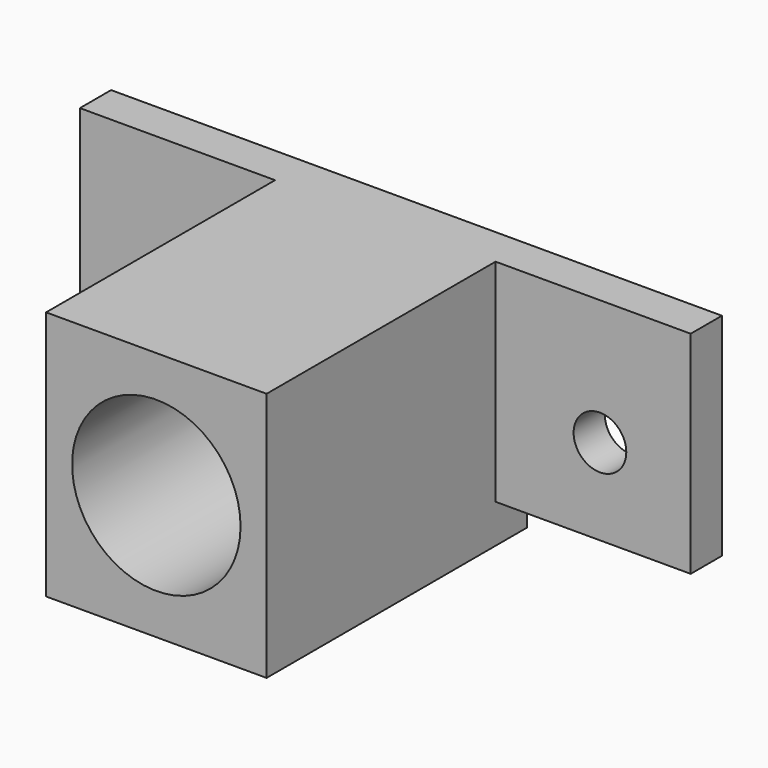
from build123d import *

# Parameters (mm, degrees)
F0_W         = 17.2212
F0_H         = 19.5351538889
F0_R         = 6.5786
F1_DEPTH     = 25.4
F2_W         = 15.24
F2_H         = 16.51
F2_R         = 2.0574
F3_DEPTH     = 3.048
F4_TEXT_SIZE = 2.3282805665
F5_DEPTH     = 22.86
F6_W         = 13.208
F6_H         = 11.43
F7_DEPTH     = 10.16


# Not quite as in the source:
# - a feature names something its author has since deleted; it is built from what else it names
# - Text() gives the source's letters only with a copy of the font that has no kerning and outlines rounded to 1/6400 em; it was checked with that copy


with BuildPart() as f1:
    # F0 (on Front) → F1 (new body)
    with BuildSketch(Plane.XZ):
        with Locations((-32.2175832933, 21.9545621703)):
            Rectangle(F0_W, F0_H)
        with Locations((-32.2175832933, 21.9405852258)):
            Circle(F0_R, mode=Mode.SUBTRACT)
    extrude(amount=F1_DEPTH)

    # F2 (on Front) → F3 (join)
    with BuildSketch(Plane.XZ):
        with Locations((-15.9869832933, 23.4671391147)):
            Rectangle(F2_W, F2_H)
        with Locations((-15.4535832933, 21.9405852258)):
            Circle(F2_R, mode=Mode.SUBTRACT)
        with Locations((-48.4481832933, 23.4671391147)):
            Rectangle(F2_W, F2_H)
        with Locations((-48.9815832933, 21.9405852258)):
            Circle(F2_R, mode=Mode.SUBTRACT)
    extrude(amount=F3_DEPTH)

    # F4 (on Front) → F5 (join)
    with BuildSketch(Plane.XZ):
        with Locations((-34.7727015615, 29.5575335622)):
            Text('R.P.U', F4_TEXT_SIZE, font='Open Sans', font_style=FontStyle.BOLD, text_align=(TextAlign.LEFT, TextAlign.BOTTOM))
    extrude(amount=F5_DEPTH)

    # F6 (on Front) → F7 (cut)
    with BuildSketch(Plane.XZ):
        with Locations((-32.0291832501, 22.4511391147)):
            Rectangle(F6_W, F6_H)
    extrude(amount=F7_DEPTH, mode=Mode.SUBTRACT)


solid = f1.part
